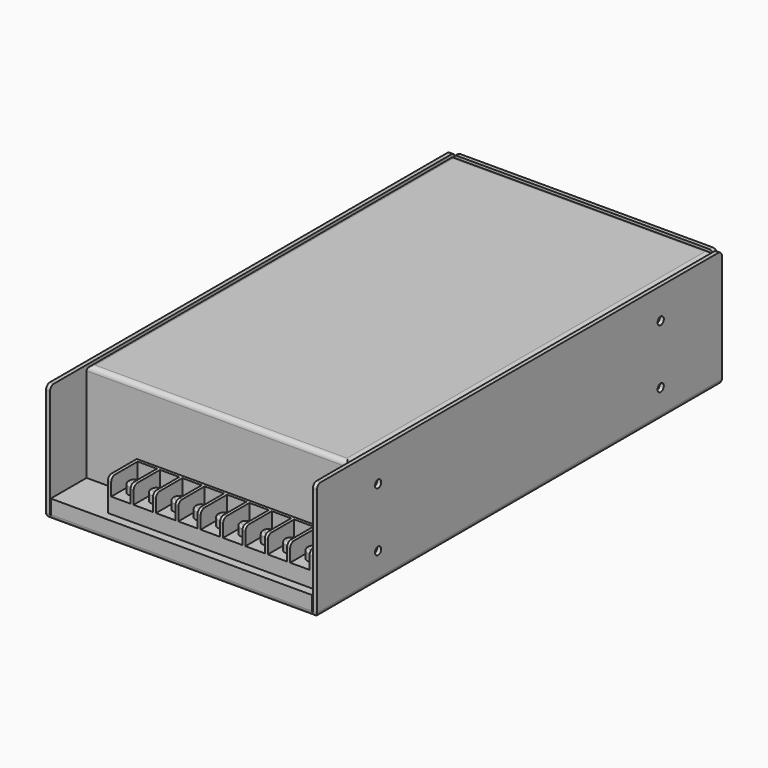
from build123d import *
from build123d import SkipClean  # not in build123d's __all__

# Parameters (mm, degrees)
F0_W             = 57.5
F0_H             = 50
F1_DEPTH         = 107.5
F2_W             = 55.8
F2_H             = 19
F3_DEPTH         = 42
F4_W             = 0.3
F4_H             = 19
F5_DEPTH         = 48.3
F6_T1_DEPTH      = 60.5
F6_T3_DEPTH      = 67.5
F6_T5_DEPTH      = 225
F6_T7_DEPTH      = 11.7
F6_T9_DEPTH      = 11.7
F6_T11_DEPTH     = 204
F6_T16_DEPTH     = 11.7
F8_W             = 87
F8_H             = 15.3
F9_DEPTH         = 14
F10_W            = 8.2
F10_H            = 14
F11_DEPTH        = 7.4
F12_T1_DEPTH     = 11.4
F12_T3_DEPTH     = 11.3
F12_T5_DEPTH     = 11.3
F12_T7_DEPTH     = 11.3
F12_T9_DEPTH     = 11.3
F12_T11_DEPTH    = 11.3
F12_T13_DEPTH    = 11.3
F12_T15_DEPTH    = 11.3
F12_T17_DEPTH    = 11.3
F12_T19_DEPTH    = 11.4
F12_2_T3_DEPTH   = 197.3
F12_2_T6_DEPTH   = 197.3
F13_R            = 2.5
F14_DEPTH        = 4
F15_R            = 1
F19_D            = 3.3
F19_DEPTH        = 5
F19_TIP          = 0.9914200214
F19_ON_F18_D     = 3.3
F19_ON_F18_DEPTH = 5
F19_ON_F18_TIP   = 0.9914200214
F19_ON_F17_D     = 3.3
F19_ON_F17_DEPTH = 5
F19_ON_F17_TIP   = 0.9914200214


# Not quite as in the source:
# - a fillet or chamfer that OpenCascade refuses, or shapes differently, is made with other operations: its cross-section is extruded or revolved along the edge and cut away or added


with BuildPart() as f1:
    # F0 (on Front) → F1 (new body, symmetric)
    with BuildSketch(Plane.XZ):
        with Locations((-28.75, 0)):
            Rectangle(F0_W, F0_H)
    extrude(amount=F1_DEPTH, both=True)

    # F2 (on face) → F3 (cut)
    with BuildSketch(Plane.XY.offset(25)):
        with Locations((-27.9, -98)):
            Rectangle(F2_W, F2_H)
    extrude(amount=-F3_DEPTH, mode=Mode.SUBTRACT)

    # F4 (on face) → F5 (cut)
    with BuildSketch(Plane.XY.offset(25)):
        Polygon((-55.8, 107.5), (-55.8, -88.5), (-55.5, -88.5), (-55.5, 105.5), (0, 105.5), (0, 105.8), (-55.5, 105.8), (-55.5, 107.5), align=None)
        with Locations((-55.65, -98)):
            Rectangle(F4_W, F4_H)
    extrude(amount=-F5_DEPTH, mode=Mode.SUBTRACT)

    # F6: fillet of radius 2 on 9 edges, made by hand

    # F6_s2 → F6_t1 (cut)
    with BuildSketch(Plane.YZ.offset(-55.5)):
        with BuildLine():
            ThreePointArc((-86.5, 25), (-87.9142135624, 24.4142135624), (-88.5, 23))
            Line((-88.5, 23), (-88.5, 25))
            Line((-88.5, 25), (-86.5, 25))
        make_face()
        with BuildLine():
            ThreePointArc((103.5, 25), (104.9142135624, 24.4142135624), (105.5, 23))
            Line((105.5, 23), (105.5, 25))
            Line((105.5, 25), (103.5, 25))
        make_face()
    extrude(amount=F6_T1_DEPTH, mode=Mode.SUBTRACT)

    # F6_s4 → F6_t3 (cut)
    with BuildSketch(Plane.YZ.offset(-62.5)):
        with BuildLine():
            ThreePointArc((-105.5, -25), (-106.9142135624, -24.4142135624), (-107.5, -23))
            Line((-107.5, -23), (-107.5, -25))
            Line((-107.5, -25), (-105.5, -25))
        make_face()
        with BuildLine():
            ThreePointArc((105.5, -25), (106.9142135624, -24.4142135624), (107.5, -23))
            Line((107.5, -23), (107.5, -25))
            Line((107.5, -25), (105.5, -25))
        make_face()
    extrude(amount=F6_T3_DEPTH, mode=Mode.SUBTRACT)

    # F6_s6 → F6_t5 (cut)
    with BuildSketch(Plane.XZ.offset(-112.5)):
        with BuildLine():
            ThreePointArc((-55.5, -25), (-56.9142135624, -24.4142135624), (-57.5, -23))
            Line((-57.5, -23), (-57.5, -25))
            Line((-57.5, -25), (-55.5, -25))
        make_face()
    extrude(amount=F6_T5_DEPTH, mode=Mode.SUBTRACT)

    # F6_s8 → F6_t7 (cut)
    with BuildSketch(Plane.YZ.offset(-62.5)):
        with BuildLine():
            ThreePointArc((-105.5, 25), (-106.9142135624, 24.4142135624), (-107.5, 23))
            Line((-107.5, 23), (-107.5, 25))
            Line((-107.5, 25), (-105.5, 25))
        make_face()
    extrude(amount=F6_T7_DEPTH, mode=Mode.SUBTRACT)

    # F6_s10 → F6_t9 (cut)
    with BuildSketch(Plane.XZ.offset(-112.5)):
        with BuildLine():
            ThreePointArc((-55.5, 23), (-54.9142135624, 24.4142135624), (-53.5, 25))
            Line((-53.5, 25), (-55.5, 25))
            Line((-55.5, 25), (-55.5, 23))
        make_face()
    extrude(amount=F6_T9_DEPTH, mode=Mode.SUBTRACT)

    # F6_s12 → F6_t11 (cut)
    with BuildSketch(Plane.XZ.offset(-110.5)):
        with BuildLine():
            ThreePointArc((-53.5, 25), (-54.9142135624, 24.4142135624), (-55.5, 23))
            Line((-55.5, 23), (-55.5, 25))
            Line((-55.5, 25), (-53.5, 25))
        make_face()
    with SkipClean():  # cleaning this boolean's faces spoils the solid; the shape is the same uncleaned
        extrude(amount=F6_T11_DEPTH, mode=Mode.SUBTRACT)


with BuildPart() as f6_tool14:
    # F6_s15 → F6_t16 (new body)
    with BuildSketch(Plane.YZ.offset(-50.8)):
        with BuildLine():
            ThreePointArc((105.5, 25), (106.9142135624, 24.4142135624), (107.5, 23))
            Line((107.5, 23), (107.5, 25))
            Line((107.5, 25), (105.5, 25))
        make_face()
    extrude(amount=-F6_T16_DEPTH)

    split(bisect_by=Plane.YZ.offset(-55.5), keep=Keep.BOTTOM)


with BuildPart() as f1_1:
    add(f1.part, clean=False)

    # F6_t13: cut F6_tool14
    add(f6_tool14.part, mode=Mode.SUBTRACT)

    # F7: F1 across plane


with BuildPart() as f1_2:
    add(f1_1.part, clean=False)
    add(f1_1.part.mirror(Plane.YZ), clean=False)

    # F12#2: fillet of radius 2 on 2 edges, made by hand


with BuildPart() as f9:
    # F8 (on face) → F9 (new body)
    with BuildSketch(Plane.XY.offset(-17)):
        with Locations((9.3, -96.15)):
            Rectangle(F8_W, F8_H)
    extrude(amount=F9_DEPTH)

    # F10 (on face) → F11 (cut)
    with BuildSketch(Plane.XY.offset(-3)):
        with Locations((-28.7, -96.8)):
            Rectangle(F10_W, F10_H)
        with Locations((-19.2, -96.8)):
            Rectangle(F10_W, F10_H)
        with Locations((-9.7, -96.8)):
            Rectangle(F10_W, F10_H)
        with Locations((-0.2, -96.8)):
            Rectangle(F10_W, F10_H)
        with Locations((9.3, -96.8)):
            Rectangle(F10_W, F10_H)
        with Locations((18.8, -96.8)):
            Rectangle(F10_W, F10_H)
        with Locations((28.3, -96.8)):
            Rectangle(F10_W, F10_H)
        with Locations((37.8, -96.8)):
            Rectangle(F10_W, F10_H)
        with Locations((47.3, -96.8)):
            Rectangle(F10_W, F10_H)
    extrude(amount=-F11_DEPTH, mode=Mode.SUBTRACT)

    # F12: fillet of radius 2 on 10 edges, made by hand

    # F12_s2 → F12_t1 (cut)
    with BuildSketch(Plane.YZ.offset(-39.2)):
        with BuildLine():
            ThreePointArc((-101.8, -3), (-103.2142135624, -3.5857864376), (-103.8, -5))
            Line((-103.8, -5), (-103.8, -3))
            Line((-103.8, -3), (-101.8, -3))
        make_face()
    extrude(amount=F12_T1_DEPTH, mode=Mode.SUBTRACT)

    # F12_s4 → F12_t3 (cut)
    with BuildSketch(Plane.YZ.offset(-29.6)):
        with BuildLine():
            ThreePointArc((-101.8, -3), (-103.2142135624, -3.5857864376), (-103.8, -5))
            Line((-103.8, -5), (-103.8, -3))
            Line((-103.8, -3), (-101.8, -3))
        make_face()
    extrude(amount=F12_T3_DEPTH, mode=Mode.SUBTRACT)

    # F12_s6 → F12_t5 (cut)
    with BuildSketch(Plane.YZ.offset(-20.1)):
        with BuildLine():
            ThreePointArc((-101.8, -3), (-103.2142135624, -3.5857864376), (-103.8, -5))
            Line((-103.8, -5), (-103.8, -3))
            Line((-103.8, -3), (-101.8, -3))
        make_face()
    extrude(amount=F12_T5_DEPTH, mode=Mode.SUBTRACT)

    # F12_s8 → F12_t7 (cut)
    with BuildSketch(Plane.YZ.offset(-10.6)):
        with BuildLine():
            ThreePointArc((-101.8, -3), (-103.2142135624, -3.5857864376), (-103.8, -5))
            Line((-103.8, -5), (-103.8, -3))
            Line((-103.8, -3), (-101.8, -3))
        make_face()
    extrude(amount=F12_T7_DEPTH, mode=Mode.SUBTRACT)

    # F12_s10 → F12_t9 (cut)
    with BuildSketch(Plane.YZ.offset(-1.1)):
        with BuildLine():
            ThreePointArc((-101.8, -3), (-103.2142135624, -3.5857864376), (-103.8, -5))
            Line((-103.8, -5), (-103.8, -3))
            Line((-103.8, -3), (-101.8, -3))
        make_face()
    extrude(amount=F12_T9_DEPTH, mode=Mode.SUBTRACT)

    # F12_s12 → F12_t11 (cut)
    with BuildSketch(Plane.YZ.offset(8.4)):
        with BuildLine():
            ThreePointArc((-101.8, -3), (-103.2142135624, -3.5857864376), (-103.8, -5))
            Line((-103.8, -5), (-103.8, -3))
            Line((-103.8, -3), (-101.8, -3))
        make_face()
    extrude(amount=F12_T11_DEPTH, mode=Mode.SUBTRACT)

    # F12_s14 → F12_t13 (cut)
    with BuildSketch(Plane.YZ.offset(17.9)):
        with BuildLine():
            ThreePointArc((-101.8, -3), (-103.2142135624, -3.5857864376), (-103.8, -5))
            Line((-103.8, -5), (-103.8, -3))
            Line((-103.8, -3), (-101.8, -3))
        make_face()
    extrude(amount=F12_T13_DEPTH, mode=Mode.SUBTRACT)

    # F12_s16 → F12_t15 (cut)
    with BuildSketch(Plane.YZ.offset(27.4)):
        with BuildLine():
            ThreePointArc((-101.8, -3), (-103.2142135624, -3.5857864376), (-103.8, -5))
            Line((-103.8, -5), (-103.8, -3))
            Line((-103.8, -3), (-101.8, -3))
        make_face()
    extrude(amount=F12_T15_DEPTH, mode=Mode.SUBTRACT)

    # F12_s18 → F12_t17 (cut)
    with BuildSketch(Plane.YZ.offset(36.9)):
        with BuildLine():
            ThreePointArc((-101.8, -3), (-103.2142135624, -3.5857864376), (-103.8, -5))
            Line((-103.8, -5), (-103.8, -3))
            Line((-103.8, -3), (-101.8, -3))
        make_face()
    extrude(amount=F12_T17_DEPTH, mode=Mode.SUBTRACT)

    # F12_s20 → F12_t19 (cut)
    with BuildSketch(Plane.YZ.offset(46.4)):
        with BuildLine():
            ThreePointArc((-101.8, -3), (-103.2142135624, -3.5857864376), (-103.8, -5))
            Line((-103.8, -5), (-103.8, -3))
            Line((-103.8, -3), (-101.8, -3))
        make_face()
    extrude(amount=F12_T19_DEPTH, mode=Mode.SUBTRACT)

    # F13 (on face) → F14 (join)
    with BuildSketch(Plane.XY.offset(-10.4)):
        with Locations((-28.7, -96.8)):
            Circle(F13_R)
        with Locations((-19.2, -96.8)):
            Circle(F13_R)
        with Locations((-9.7, -96.8)):
            Circle(F13_R)
        with Locations((-0.2, -96.8)):
            Circle(F13_R)
        with Locations((9.3, -96.8)):
            Circle(F13_R)
        with Locations((18.8, -96.8)):
            Circle(F13_R)
        with Locations((28.3, -96.8)):
            Circle(F13_R)
        with Locations((37.8, -96.8)):
            Circle(F13_R)
        with Locations((47.3, -96.8)):
            Circle(F13_R)
    extrude(amount=F14_DEPTH)

    # F15
    f15_edges = [f9.edges().sort_by_distance(p)[0] for p in [
        (-31.2, -96.8, -6.4),
        (-21.7, -96.8, -6.4),
        (-12.2, -96.8, -6.4),
        (-2.7, -96.8, -6.4),
        (6.8, -96.8, -6.4),
        (16.3, -96.8, -6.4),
        (25.8, -96.8, -6.4),
        (35.3, -96.8, -6.4),
        (44.8, -96.8, -6.4),
    ]]
    fillet(f15_edges, radius=F15_R)


with BuildPart() as f12_2_tool1:
    # F12_2_s2 → F12_2_t3 (new body)
    with BuildSketch(Plane.XZ.offset(91.5)):
        with BuildLine():
            ThreePointArc((-53.5, 25), (-54.9142135624, 24.4142135624), (-55.5, 23))
            Line((-55.5, 23), (-55.5, 25))
            Line((-55.5, 25), (-53.5, 25))
        make_face()
    extrude(amount=-F12_2_T3_DEPTH)


with BuildPart() as f12_2_tool4:
    # F12_2_s5 → F12_2_t6 (new body)
    with BuildSketch(Plane.XZ.offset(91.5)):
        with BuildLine():
            ThreePointArc((53.5, 25), (54.9142135624, 24.4142135624), (55.5, 23))
            Line((55.5, 23), (55.5, 25))
            Line((55.5, 25), (53.5, 25))
        make_face()
    extrude(amount=-F12_2_T6_DEPTH)


with BuildPart() as f1_3:
    add(f1_2.part, clean=False)

    # F12_2_t7: cut F12_2_tool1, F12_2_tool4
    add([f12_2_tool1.part, f12_2_tool4.part], mode=Mode.SUBTRACT)

    # F19
    with Locations(Plane(origin=(-57.5, 0, 0), x_dir=(0, -1, 0), z_dir=(-1, 0, 0))):
        with Locations((-75, -13), (75, -13)):
            Hole(F19_D / 2, depth=F19_DEPTH)
            with Locations((0, 0, -(F19_DEPTH + F19_TIP / 2))):  # 118° drill point
                Cone(0, F19_D / 2, F19_TIP, mode=Mode.SUBTRACT)

    # F19 on F18
    with Locations(Plane(origin=(0, 0, -25), x_dir=(1, 0, 0), z_dir=(0, 0, -1))):
        with Locations((-25, -75), (-25, 75), (25, -75), (25, 75)):
            Hole(F19_ON_F18_D / 2, depth=F19_ON_F18_DEPTH)
            with Locations((0, 0, -(F19_ON_F18_DEPTH + F19_ON_F18_TIP / 2))):  # 118° drill point
                Cone(0, F19_ON_F18_D / 2, F19_ON_F18_TIP, mode=Mode.SUBTRACT)

    # F19 on F17
    with Locations(Plane.YZ.offset(57.5)):
        with Locations((-75, -13), (-75, 12), (75, 12), (75, -13)):
            Hole(F19_ON_F17_D / 2, depth=F19_ON_F17_DEPTH)
            with Locations((0, 0, -(F19_ON_F17_DEPTH + F19_ON_F17_TIP / 2))):  # 118° drill point
                Cone(0, F19_ON_F17_D / 2, F19_ON_F17_TIP, mode=Mode.SUBTRACT)


solid = Compound([f9.part, f1_3.part])
